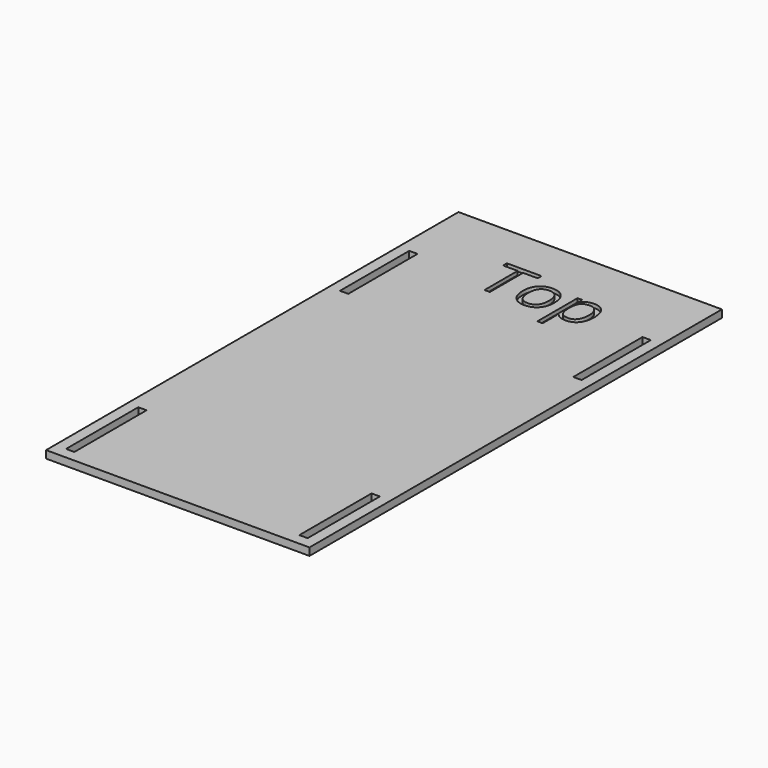
from build123d import *

# Parameters (mm, degrees)
F0_W         = 70
F0_H         = 137
F1_DEPTH     = 2
F2_W         = 2.2
F2_H         = 23
F2_H_2       = 24
F3_DEPTH     = 25
F4_TEXT_SIZE = 17.2111981859
F5_DEPTH     = 1


# Not quite as in the source:
# - Text() gives the source's letters only with a copy of the font that has no kerning and outlines rounded to 1/6400 em; it was checked with that copy


with BuildPart() as f1:
    # F0 (on Top) → F1 (new body)
    with BuildSketch(Plane.XY):
        with Locations((-1.4516115189, 14.1015607945)):
            Rectangle(F0_W, F0_H)
    extrude(amount=F1_DEPTH)

    # F2 (on Top) → F3 (cut)
    with BuildSketch(Plane.XY):
        with Locations((-32.4516115189, 51.1015607945)):
            Rectangle(F2_W, F2_H)
        with Locations((29.5483884811, 51.1015607945)):
            Rectangle(F2_W, F2_H)
        with Locations((-32.4516115189, -39.3984392055)):
            Rectangle(F2_W, F2_H_2)
        with Locations((29.5483884811, -39.3984392055)):
            Rectangle(F2_W, F2_H_2)
    extrude(amount=F3_DEPTH, mode=Mode.SUBTRACT)

    # F4 (on face) → F5 (cut)
    with BuildSketch(Plane.XY.offset(2)):
        with Locations((-14.3938522669, 58.6118064821)):
            Text('Top', F4_TEXT_SIZE, font='Open Sans', text_align=(TextAlign.LEFT, TextAlign.BOTTOM))
    extrude(amount=-F5_DEPTH, mode=Mode.SUBTRACT)


solid = f1.part
